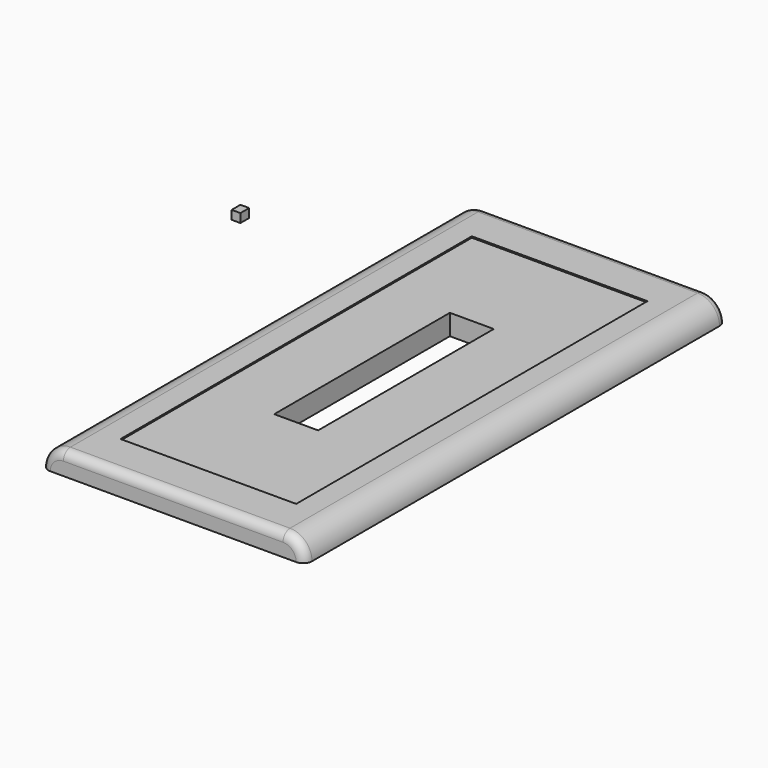
from build123d import *

# Parameters (mm, degrees)
F0_W         = 60
F0_H         = 120
F0_W_2       = 40
F0_H_2       = 100
F1_DEPTH     = 5
F2_R         = 4.99999
F3_T1_DEPTH  = 50.00002
F3_T3_DEPTH  = 5.00001
F3_T6_ANGLE  = 90
F3_T8_ANGLE  = 90
F3_T10_ANGLE = 90
F3_T12_ANGLE = 90
F0_W_3       = 10
F0_H_3       = 50
F4_DEPTH     = 4.7
F5_W         = 2
F5_H         = 2.5
F6_DEPTH     = 2


# Not quite as in the source:
# - a fillet or chamfer that OpenCascade refuses, or shapes differently, is made with other operations: its cross-section is extruded or revolved along the edge and cut away or added
# - a fillet or chamfer is up to 0.001 mm smaller than in the source, because OpenCascade refuses the exact size


with BuildPart() as f1:
    # F0 (on Top) → F1 (new body)
    with BuildSketch(Plane.XY):
        Rectangle(F0_W, F0_H)
        Rectangle(F0_W_2, F0_H_2, mode=Mode.SUBTRACT)
    extrude(amount=F1_DEPTH)

    # F2 (radius 5 in the source; OpenCascade refuses exactly that, so slightly less here)
    f2_edges = [f1.edges().sort_by_distance(p)[0] for p in [
        (-30, 0, 5),
        (30, 0, 5),
    ]]
    fillet(f2_edges, radius=F2_R)

    # F3: fillet of radius 2 on 2 edges, made by hand

    # F3_s2 → F3_t1 (cut)
    with BuildSketch(Plane.YZ.offset(-25.00001)):
        with BuildLine():
            ThreePointArc((60, 3), (59.4142135624, 4.4142135624), (58, 5))
            Line((58, 5), (60, 5))
            Line((60, 5), (60, 3))
        make_face()
        with BuildLine():
            ThreePointArc((-58, 5), (-59.4142135624, 4.4142135624), (-60, 3))
            Line((-60, 3), (-60, 5))
            Line((-60, 5), (-58, 5))
        make_face()
    extrude(amount=F3_T1_DEPTH, mode=Mode.SUBTRACT)

    # F3_s4 → F3_t3 (cut)
    with BuildSketch(Plane.XY.offset(-5)):
        with BuildLine():
            ThreePointArc((30, -58), (29.4142135624, -59.4142135624), (28, -60))
            Line((28, -60), (30, -60))
            Line((30, -60), (30, -58))
        make_face()
        with BuildLine():
            ThreePointArc((-30, -58), (-29.4142135624, -59.4142135624), (-28, -60))
            Line((-28, -60), (-30, -60))
            Line((-30, -60), (-30, -58))
        make_face()
        with BuildLine():
            ThreePointArc((-28, 60), (-29.4142135624, 59.4142135624), (-30, 58))
            Line((-30, 58), (-30, 60))
            Line((-30, 60), (-28, 60))
        make_face()
        with BuildLine():
            ThreePointArc((28, 60), (29.4142135624, 59.4142135624), (30, 58))
            Line((30, 58), (30, 60))
            Line((30, 60), (28, 60))
        make_face()
    extrude(amount=F3_T3_DEPTH, mode=Mode.SUBTRACT)

    # F3_s5 → F3_t6 (revolve, cut)
    with BuildSketch(Plane.XY.offset(1e-05)):
        with BuildLine():
            ThreePointArc((-30, -58), (-29.4142135624, -59.4142135624), (-28, -60))
            Line((-28, -60), (-30, -60))
            Line((-30, -60), (-30, -58))
        make_face()
    revolve(axis=Axis((-25.00001, -60, 1e-05), (0, 1, 0)), revolution_arc=F3_T6_ANGLE, mode=Mode.SUBTRACT)

    # F3_s7 → F3_t8 (revolve, cut)
    with BuildSketch(Plane.XY.offset(1e-05)):
        with BuildLine():
            ThreePointArc((30, -58), (29.4142135624, -59.4142135624), (28, -60))
            Line((28, -60), (30, -60))
            Line((30, -60), (30, -58))
        make_face()
    revolve(axis=Axis((25.00001, -60, 1e-05), (0, -1, 0)), revolution_arc=F3_T8_ANGLE, mode=Mode.SUBTRACT)

    # F3_s9 → F3_t10 (revolve, cut)
    with BuildSketch(Plane.XY.offset(1e-05)):
        with BuildLine():
            ThreePointArc((28, 60), (29.4142135624, 59.4142135624), (30, 58))
            Line((30, 58), (30, 60))
            Line((30, 60), (28, 60))
        make_face()
    revolve(axis=Axis((25.00001, 60, 1e-05), (0, -1, 0)), revolution_arc=F3_T10_ANGLE, mode=Mode.SUBTRACT)

    # F3_s11 → F3_t12 (revolve, cut)
    with BuildSketch(Plane.XY.offset(1e-05)):
        with BuildLine():
            ThreePointArc((-28, 60), (-29.4142135624, 59.4142135624), (-30, 58))
            Line((-30, 58), (-30, 60))
            Line((-30, 60), (-28, 60))
        make_face()
    revolve(axis=Axis((-25.00001, 60, 1e-05), (0, 1, 0)), revolution_arc=F3_T12_ANGLE, mode=Mode.SUBTRACT)

    # F0 (on Top) → F4 (join)
    with BuildSketch(Plane.XY):
        Rectangle(F0_W_2, F0_H_2)
        Rectangle(F0_W_3, F0_H_3, mode=Mode.SUBTRACT)
    extrude(amount=F4_DEPTH)


with BuildPart() as f6:
    # F5 (on Top) → F6 (new body)
    with BuildSketch(Plane.XY):
        with Locations((-62.3082230687, 37.0115598826)):
            Rectangle(F5_W, F5_H)
    extrude(amount=F6_DEPTH)


solid = Compound([f1.part, f6.part])
